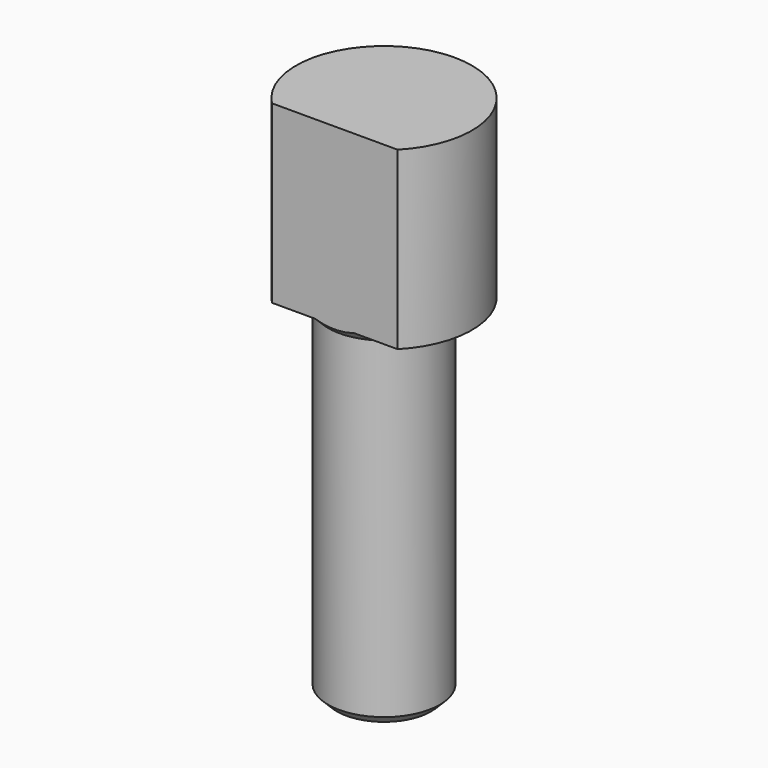
from build123d import *

# Parameters (mm, degrees)
F0_R     = 8.0772
F1_DEPTH = 50.48541
F2_R     = 12.7227956512
F3_DEPTH = 25.4
F5_DEPTH = 25.4


# Not quite as in the source:
# - a fillet or chamfer that OpenCascade refuses, or shapes differently, is made with other operations: its cross-section is extruded or revolved along the edge and cut away or added


with BuildPart() as f1:
    # F0 (on Top) → F1 (new body)
    with BuildSketch(Plane.XY):
        Circle(F0_R)
    extrude(amount=F1_DEPTH)

    # F2 (on face) → F3 (join)
    with BuildSketch(Plane.XY.offset(50.48541)):
        Circle(F2_R)
    extrude(amount=F3_DEPTH)

    # F4 (on face) → F5 (cut)
    with BuildSketch(Plane.XY.offset(75.88541)):
        with BuildLine():
            Line((9.0839408688, -8.9079485558), (-9.0839408688, -8.9079485558))
            ThreePointArc((-9.0839408688, -8.9079485558), (0, -12.7227956512), (9.0839408688, -8.9079485558))
        make_face()
    extrude(amount=-F5_DEPTH, mode=Mode.SUBTRACT)

    # F6: chamfer of 1.27 on 2 edges, made by hand


with BuildPart() as f6_tool2:
    # F6_s3 → F6_t4 (revolve)
    with BuildSketch(Plane.XZ):
        Polygon((9.3472, 50.48541), (8.0772, 49.21541), (8.0772, 50.48541), align=None)
    revolve(axis=Axis((0, 0, 50.48541), (0, 0, 1)))

    split(bisect_by=Plane.XZ.offset(8.9079485558), keep=Keep.BOTTOM)


with BuildPart() as f1_1:
    add(f1.part)

    # F6_t1: union F6_tool2
    add(f6_tool2.part)

    # F6_s6 → F6_t7 (revolve, cut)
    with BuildSketch(Plane.XZ):
        Polygon((8.0772, 1.27), (6.8072, 0), (8.0772, 0), align=None)
    revolve(axis=Axis((0, 0, 0), (0, 0, 1)), mode=Mode.SUBTRACT)


solid = f1_1.part
